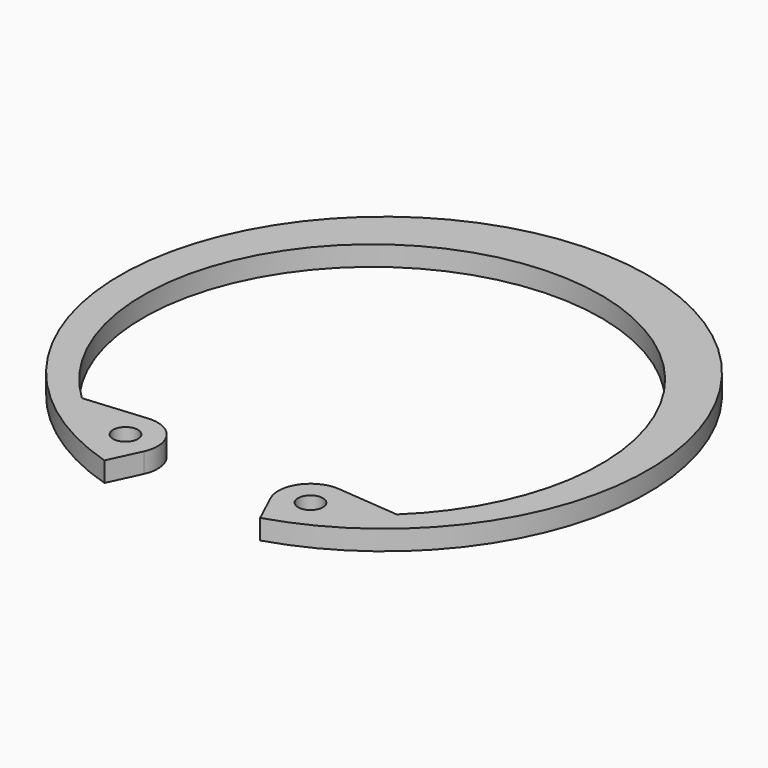
from build123d import *

# Parameters (mm, degrees)
F0_R     = 0.9906
F1_DEPTH = 1.5875


# Not quite as in the source:
# - ends of sketch curves that miss each other by under 0.0002 mm in the source are joined


with BuildPart() as f1:
    # F0 (on Top) → F1 (new body)
    with BuildSketch(Plane.XY):
        with BuildLine():
            Line((41.6924998, -18.8505592), (42.8484792, -21.3295484))
            ThreePointArc((42.8484792, -21.3295484), (36.6378236, 19.8468996), (30.4271688612, -21.32954561))
            Line((30.4271688612, -21.32954561), (31.5831474, -18.8505592))
            ThreePointArc((31.5831474, -18.8505592), (31.3595624423, -16.2949103348), (29.034512192, -15.2107228522))
            Line((29.034512192, -15.2107228522), (24.075517, -15.6445712))
            ThreePointArc((24.075517, -15.6445712), (36.6378236, 15.8590996), (49.2001483474, -15.6445903367))
            Line((49.2001483474, -15.6445903367), (44.2411358, -15.2107138))
            ThreePointArc((44.2411358, -15.2107138), (41.9160847577, -16.2949103348), (41.6924998, -18.8505592))
        make_face()
        with Locations((29.2581076, -17.7663602)):
            Circle(F0_R, mode=Mode.SUBTRACT)
        with Locations((44.0175396, -17.7663602)):
            Circle(F0_R, mode=Mode.SUBTRACT)
    extrude(amount=-F1_DEPTH)


with BuildPart() as f1_1:
    # F3: moved
    add(f1.part.moved(Location((-36.6378236, -19.8468996, 0))))


with BuildPart() as f1_2:
    # F4: moved
    add(f1_1.part.moved(Location((0, 21.0566, 0))))


solid = f1_2.part
